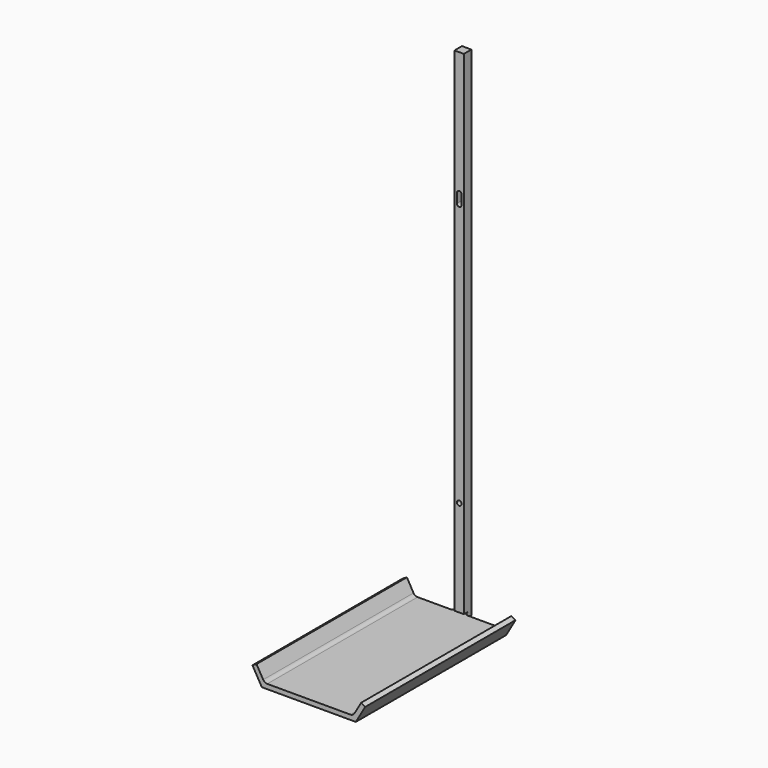
from build123d import *

# Parameters (mm, degrees)
F1_DEPTH = 200
F2_W     = 10
F2_H     = 530
F2_R     = 2.5
F3_DEPTH = 10
F4_R     = 5


with BuildPart() as f1:
    # F0 (on Front) → F1 (new body)
    with BuildSketch(Plane.XZ):
        Polygon((-60, 17.3205080757), (-50, 0), (0, 0), (50, 0), (60, 17.3205080757), (55.6698729811, 19.8205080757), (47.1132486541, 5), (0, 5), (-47.1132486541, 5), (-55.6698729811, 19.8205080757), align=None)
    extrude(amount=F1_DEPTH)

    # F2 (on Front) → F3 (join)
    with BuildSketch(Plane.XZ):
        with Locations((0, 265)):
            Rectangle(F2_W, F2_H)
        with Locations((0, 107.5)):
            Circle(F2_R, mode=Mode.SUBTRACT)
        with BuildLine():
            ThreePointArc((-2.5, 397.5), (0, 400), (2.5, 397.5))
            Line((2.5, 397.5), (2.5, 387.5))
            ThreePointArc((2.5, 387.5), (0, 385), (-2.5, 387.5))
            Line((-2.5, 387.5), (-2.5, 397.5))
        make_face(mode=Mode.SUBTRACT)
    extrude(amount=-F3_DEPTH)

    # F4
    f4_edges = [f1.edges().sort_by_distance(p)[0] for p in [
        (47.113249, -100, 5),
        (-47.113249, -100, 5),
        (5, 0, 2.5),
        (-5, 0, 2.5),
    ]]
    fillet(f4_edges, radius=F4_R)


solid = f1.part
